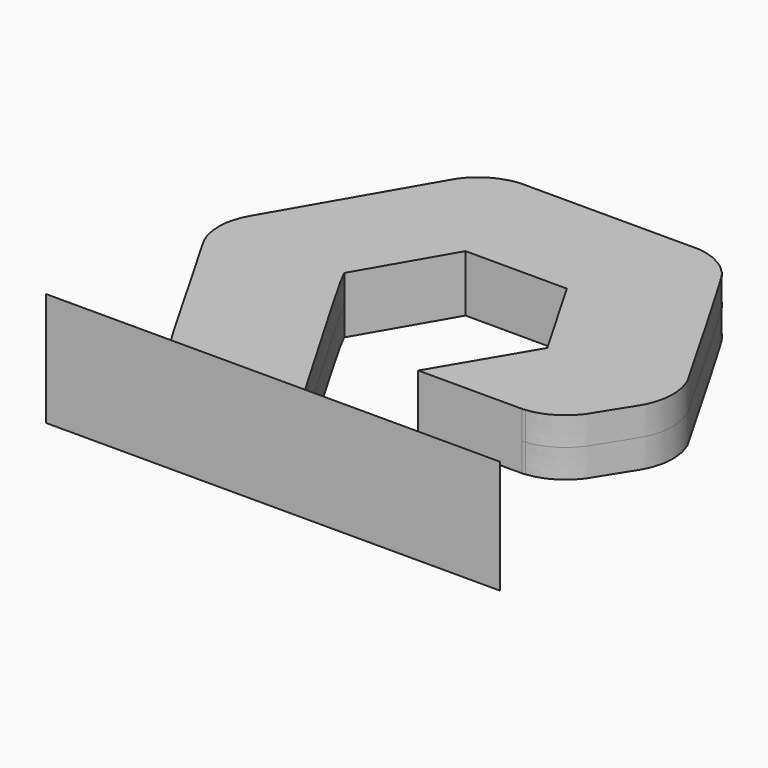
from build123d import *

# Parameters (mm, degrees)
F1_DEPTH    = 3.175
F2_DEPTH    = 1.5875
F3_DEPTH    = 1.5875
F4_T1_DEPTH = 22.6801869736
F4_T3_DEPTH = 41.7253830583


# Not quite as in the source:
# - a fillet or chamfer that OpenCascade refuses, or shapes differently, is made with other operations: its cross-section is extruded or revolved along the edge and cut away or added


with BuildPart() as f1:
    # F0 (on Top) → F1 (new body, symmetric)
    with BuildSketch(Plane.XY):
        with BuildLine():
            add(Edge.make_bspline(
                [(-8.0979492671, -8.4599665572), (-7.8144543772, -8.9512922446), (-7.4012331652, -9.6478596679), (-7.2094447017, -9.853233929), (-7.0198074368, -10.0624663427), (-6.8247908118, -10.2363901293), (-6.6355575508, -10.3900701529), (-6.4438841868, -10.5234739102), (-6.0350828964, -10.7264789939), (-5.8763022274, -10.78836422), (-5.4940772788, -10.9232334645), (-5.1611591338, -10.9716922009), (-4.9454318311, -10.9894729499), (-4.8368193396, -10.9980083466), (-1.8185705834, -10.9990381649), (0.9024133324, -10.9999665572)],
                knots=[0.5399683447, 0.5399683447, 0.5399683447, 0.5399683447, 0.583735527, 0.615598334, 0.6417416026, 0.6683965868, 0.6934366825, 0.7191935337, 0.7535274628, 0.7758085206, 0.8081226598, 0.8394404995, 0.861841058, 0.8754482187, 1, 1, 1, 1], degree=3))
            Line((-8.0979492671, -8.4599665572), (-12.7, -8.4599665572))
            Line((-12.7, -8.4599665572), (-12.7, -11.6349665572))
            Line((-12.7, -11.6349665572), (12.6951960847, -11.6349665572))
            Line((12.6951960847, -11.6349665572), (12.6951960847, -8.4599665572))
            Line((12.6951960847, -8.4599665572), (-0.5820742577, -8.4599665572))
            add(Edge.make_bspline(
                [(-0.5820742577, -8.4599665572), (-0.0948763272, -9.2939885426), (0.4037685026, -10.1469775499), (0.9024133324, -10.9999665572)],
                knots=[0.8523529488, 0.8523529488, 0.8523529488, 0.8523529488, 1, 1, 1, 1], degree=3))
        make_face()
        with BuildLine():
            Line((-0.5820742577, -8.4599665572), (-8.0979492671, -8.4599665572))
            add(Edge.make_bspline(
                [(-8.0979492671, -8.4599665572), (-7.8144543772, -8.9512922446), (-7.4012331652, -9.6478596679), (-7.2094447017, -9.853233929), (-7.0198074368, -10.0624663427), (-6.8247908118, -10.2363901293), (-6.6355575508, -10.3900701529), (-6.4438841868, -10.5234739102), (-6.0350828964, -10.7264789939), (-5.8763022274, -10.78836422), (-5.4940772788, -10.9232334645), (-5.1611591338, -10.9716922009), (-4.9454318311, -10.9894729499), (-4.8368193396, -10.9980083466), (-1.8185705834, -10.9990381649), (0.9024133324, -10.9999665572)],
                knots=[0.5399683447, 0.5399683447, 0.5399683447, 0.5399683447, 0.583735527, 0.615598334, 0.6417416026, 0.6683965868, 0.6934366825, 0.7191935337, 0.7535274628, 0.7758085206, 0.8081226598, 0.8394404995, 0.861841058, 0.8754482187, 1, 1, 1, 1], degree=3))
            add(Edge.make_bspline(
                [(-0.5820742577, -8.4599665572), (-0.0948763272, -9.2939885426), (0.4037685026, -10.1469775499), (0.9024133324, -10.9999665572)],
                knots=[0.8523529488, 0.8523529488, 0.8523529488, 0.8523529488, 1, 1, 1, 1], degree=3))
        make_face()
    extrude(amount=F1_DEPTH, both=True)

    # F0 (on Top) → F2 (cut, symmetric)
    with BuildSketch(Plane.XY):
        with BuildLine():
            add(Edge.make_bspline(
                [(-4.9467352219, 11.8727972619), (-2.6941970372, 11.8727972619), (-0.4416588525, 11.8727972619), (1.8108793323, 11.8727972619)],
                knots=[0.5524163134, 0.5524163134, 0.5524163134, 0.5524163134, 7.3100308676, 7.3100308676, 7.3100308676, 7.3100308676], degree=3))
            add(Edge.make_bspline(
                [(-12.1819954365, 2.2322773002), (-10.2153621206, 5.6292283823), (-7.918654142, 9.5963149713), (-7.7561059918, 9.8938723276), (-7.595936966, 10.1748103574), (-7.4488921306, 10.429639936), (-7.2380091716, 10.7143793357), (-7.0022497381, 10.9732635429), (-6.7468930063, 11.1814042046), (-6.6123462397, 11.2802086076), (-6.44534623, 11.390971666), (-6.3180815613, 11.463666659), (-6.1526142879, 11.5500745414), (-6.0434056072, 11.6051608595), (-5.8991320293, 11.660363592), (-5.6381957934, 11.7542790581), (-5.4211920209, 11.8110346891), (-5.1249038455, 11.8530818861), (-5.1009011539, 11.8676549492), (-4.9467352219, 11.8727972619)],
                knots=[0, 0, 0, 0, 0.1520022985, 0.1775139721, 0.2052814017, 0.2338919375, 0.2644870562, 0.2956347735, 0.3249719317, 0.3463123249, 0.3689682109, 0.3892301717, 0.411329997, 0.4293235674, 0.449497138, 0.4765503291, 0.5022012755, 0.5278147587, 0.5520405652, 0.5520405652, 0.5520405652, 0.5520405652], degree=3))
            add(Edge.make_bspline(
                [(-12.1819954365, 2.2322773002), (-12.2139037883, 2.1703194424), (-12.283482926, 2.0352145533), (-12.4406884255, 1.7801306072), (-12.6198918883, 1.2441500466), (-12.7164267868, 0.7551726738), (-12.7062312963, 0.3123164438), (-12.6510102494, -0.2863243011), (-12.5128439568, -0.6906531958), (-12.348735221, -1.0976190794), (-11.6470462247, -2.2552827891), (-11.0471565611, -3.3365181876), (-9.6670924889, -5.6885534643), (-8.4674528036, -7.819579074), (-8.0979492671, -8.4599665572)],
                knots=[0, 0, 0, 0, 0.0239021006, 0.0521207603, 0.0910959498, 0.1277402468, 0.1623042864, 0.2023672629, 0.23552051, 0.2695660314, 0.3281617082, 0.3861383143, 0.4829227709, 0.5399683447, 0.5399683447, 0.5399683447, 0.5399683447], degree=3))
            Line((-8.0979492671, -8.4599665572), (-0.5820742577, -8.4599665572))
            add(Edge.make_bspline(
                [(-5.6781647727, 0.4474149318), (-5.6798237666, 0.4432516249), (-5.716895521, 0.3502186819), (-3.2687593621, -3.8606973389), (-0.5820742577, -8.4599665572)],
                knots=[0, 0, 0, 0, 0.0381435521, 0.8523529488, 0.8523529488, 0.8523529488, 0.8523529488], degree=3))
            add(Edge.make_bspline(
                [(-2.836742904, 5.3628673777), (-3.7838835269, 3.7243832291), (-4.7310241498, 2.0858990805), (-5.6781647727, 0.4474149318)],
                knots=[0, 0, 0, 0, 5.6776184253, 5.6776184253, 5.6776184253, 5.6776184253], degree=3))
            add(Edge.make_bspline(
                [(2.8362337034, 5.3595150821), (0.9452415009, 5.360632514), (-0.9457507016, 5.3617499458), (-2.836742904, 5.3628673777)],
                knots=[0, 0, 0, 0, 5.6729775979, 5.6729775979, 5.6729775979, 5.6729775979], degree=3))
            add(Edge.make_bspline(
                [(5.6763379835, 0.4443899379), (4.7296365568, 2.082764986), (3.7829351301, 3.721140034), (2.8362337034, 5.3595150821)],
                knots=[0, 0, 0, 0, 5.6766757442, 5.6766757442, 5.6766757442, 5.6766757442], degree=3))
            add(Edge.make_bspline(
                [(2.6081528049, -4.7463672236), (3.6308811978, -3.0161148364), (4.6536095906, -1.2858624492), (5.6763379835, 0.4443899379)],
                knots=[0, 0, 0, 0, 6.0297363292, 6.0297363292, 6.0297363292, 6.0297363292], degree=3))
            Line((2.6081528049, -4.7463672236), (8.3983913064, -4.7463672236))
            add(Edge.make_bspline(
                [(8.3983913064, -4.7463672236), (8.4285802649, -4.7476342502), (8.4896773359, -4.7501984863), (8.5516653278, -4.7371940519), (8.5830241442, -4.7306152992)],
                knots=[0, 0, 0, 0, 0.4941146609, 1, 1, 1, 1], degree=3))
            add(Edge.make_bspline(
                [(7.394594606, 10.4755461216), (7.4049946498, 10.4644086633), (7.4978359113, 10.3649844979), (12.37583426, 1.9246802289), (12.3732313137, 1.8788009391), (12.4554314204, 1.7100351498), (12.5092309984, 1.5407375676), (12.579223391, 1.3481749221), (12.6327811924, 1.1548508933), (12.6617328431, 0.9474132467), (12.6887145756, 0.7331187902), (12.7057320419, 0.4773166934), (12.6885501549, 0.1892988959), (12.6579644324, -0.1503660031), (12.6047454763, -0.3551130001), (12.5476882015, -0.5689364186), (12.4644072913, -0.7996513773), (12.3592844301, -1.0395808564), (12.2025247276, -1.3122675142), (11.5798542764, -2.2842021351), (11.0022863487, -3.2119016224), (10.8931559285, -3.3988812592), (10.7117863794, -3.6224692911), (10.497630846, -3.8442513774), (10.2817003921, -4.0291717223), (10.0560553294, -4.2067210739), (9.8433649464, -4.3187164368), (9.7865197525, -4.3546553415), (9.5130416542, -4.505924573), (9.2077822138, -4.5905623978), (9.0144989656, -4.6706733119), (8.6495598585, -4.7218623963), (8.5981329416, -4.7286277074), (8.5830241442, -4.7306152992)],
                knots=[0, 0, 0, 0, 0.0211617068, 0.1889107002, 0.2086954298, 0.2296465529, 0.2530764843, 0.2773859957, 0.3015816681, 0.3261482383, 0.3512044462, 0.3783001026, 0.40768826, 0.4390979831, 0.4639315394, 0.4889953709, 0.5158573886, 0.5426802508, 0.5721507083, 0.6312181763, 0.6877344447, 0.7121562897, 0.7402266081, 0.7704940169, 0.7992541414, 0.828820597, 0.8543275782, 0.8684516809, 0.8979328023, 0.9286239977, 0.9544581079, 0.9866201736, 1, 1, 1, 1], degree=3))
            add(Edge.make_bspline(
                [(5.0841737539, 11.8727972619), (5.1354007842, 11.8660248609), (5.285102127, 11.8344246259), (5.511192311, 11.7972110307), (5.856974007, 11.6822825291), (6.0571511062, 11.6028524692), (6.5572225021, 11.3301125557), (6.8102335511, 11.1329565648), (7.0714115659, 10.8810767284), (7.2647332021, 10.6836819238), (7.3523685742, 10.5432240362), (7.394594606, 10.4755461216)],
                knots=[0.7441231562, 0.7441231562, 0.7441231562, 0.7441231562, 0.7668331465, 0.7924407066, 0.8229285687, 0.8479598314, 0.8863005426, 0.9166541286, 0.9473218688, 0.974617687, 1, 1, 1, 1], degree=3))
            add(Edge.make_bspline(
                [(4.7206622548, 11.8727972619), (4.8418327545, 11.8727972619), (4.9630032542, 11.8727972619), (5.0841737539, 11.8727972619)],
                knots=[10.2198137902, 10.2198137902, 10.2198137902, 10.2198137902, 10.5833252892, 10.5833252892, 10.5833252892, 10.5833252892], degree=3))
            add(Edge.make_bspline(
                [(1.8108793323, 11.8727972619), (3.1458171486, 11.8689304093), (4.2714307431, 11.8669693291), (4.7206622548, 11.8727972619)],
                knots=[0.6587883417, 0.6587883417, 0.6587883417, 0.6587883417, 0.7129256384, 0.7129256384, 0.7129256384, 0.7129256384], degree=3))
        make_face()
        with BuildLine():
            Line((-0.5820742577, -8.4599665572), (-8.0979492671, -8.4599665572))
            add(Edge.make_bspline(
                [(-8.0979492671, -8.4599665572), (-7.8144543772, -8.9512922446), (-7.4012331652, -9.6478596679), (-7.2094447017, -9.853233929), (-7.0198074368, -10.0624663427), (-6.8247908118, -10.2363901293), (-6.6355575508, -10.3900701529), (-6.4438841868, -10.5234739102), (-6.0350828964, -10.7264789939), (-5.8763022274, -10.78836422), (-5.4940772788, -10.9232334645), (-5.1611591338, -10.9716922009), (-4.9454318311, -10.9894729499), (-4.8368193396, -10.9980083466), (-1.8185705834, -10.9990381649), (0.9024133324, -10.9999665572)],
                knots=[0.5399683447, 0.5399683447, 0.5399683447, 0.5399683447, 0.583735527, 0.615598334, 0.6417416026, 0.6683965868, 0.6934366825, 0.7191935337, 0.7535274628, 0.7758085206, 0.8081226598, 0.8394404995, 0.861841058, 0.8754482187, 1, 1, 1, 1], degree=3))
            add(Edge.make_bspline(
                [(-0.5820742577, -8.4599665572), (-0.0948763272, -9.2939885426), (0.4037685026, -10.1469775499), (0.9024133324, -10.9999665572)],
                knots=[0.8523529488, 0.8523529488, 0.8523529488, 0.8523529488, 1, 1, 1, 1], degree=3))
        make_face()
    extrude(amount=F2_DEPTH, both=True, mode=Mode.SUBTRACT)

    # F4: chamfer of 3.175 on 4 edges, made by hand

    # F4_s2 → F4_t1 (cut)
    with BuildSketch(Plane.XY.offset(-11.3400934868)):
        Polygon((-9.525, -8.4599665572), (-12.7, -11.6349665572), (-12.7, -8.4599665572), align=None)
        Polygon((9.5201960847, -8.4599665572), (12.6951960847, -11.6349665572), (12.6951960847, -8.4599665572), align=None)
    extrude(amount=F4_T1_DEPTH, mode=Mode.SUBTRACT)

    # F4_s4 → F4_t3 (cut)
    with BuildSketch(Plane.YZ.offset(-20.8650934868)):
        Polygon((-8.4599665572, 0), (-11.6349665572, 3.175), (-8.4599665572, 3.175), align=None)
        Polygon((-8.4599665572, 0), (-11.6349665572, -3.175), (-8.4599665572, -3.175), align=None)
    extrude(amount=F4_T3_DEPTH, mode=Mode.SUBTRACT)


with BuildPart() as f3:
    # F0 (on Top) → F3 (new body, symmetric)
    with BuildSketch(Plane.XY):
        with BuildLine():
            add(Edge.make_bspline(
                [(-4.9467352219, 11.8727972619), (-2.6941970372, 11.8727972619), (-0.4416588525, 11.8727972619), (1.8108793323, 11.8727972619)],
                knots=[0.5524163134, 0.5524163134, 0.5524163134, 0.5524163134, 7.3100308676, 7.3100308676, 7.3100308676, 7.3100308676], degree=3))
            add(Edge.make_bspline(
                [(-12.1819954365, 2.2322773002), (-10.2153621206, 5.6292283823), (-7.918654142, 9.5963149713), (-7.7561059918, 9.8938723276), (-7.595936966, 10.1748103574), (-7.4488921306, 10.429639936), (-7.2380091716, 10.7143793357), (-7.0022497381, 10.9732635429), (-6.7468930063, 11.1814042046), (-6.6123462397, 11.2802086076), (-6.44534623, 11.390971666), (-6.3180815613, 11.463666659), (-6.1526142879, 11.5500745414), (-6.0434056072, 11.6051608595), (-5.8991320293, 11.660363592), (-5.6381957934, 11.7542790581), (-5.4211920209, 11.8110346891), (-5.1249038455, 11.8530818861), (-5.1009011539, 11.8676549492), (-4.9467352219, 11.8727972619)],
                knots=[0, 0, 0, 0, 0.1520022985, 0.1775139721, 0.2052814017, 0.2338919375, 0.2644870562, 0.2956347735, 0.3249719317, 0.3463123249, 0.3689682109, 0.3892301717, 0.411329997, 0.4293235674, 0.449497138, 0.4765503291, 0.5022012755, 0.5278147587, 0.5520405652, 0.5520405652, 0.5520405652, 0.5520405652], degree=3))
            add(Edge.make_bspline(
                [(-12.1819954365, 2.2322773002), (-12.2139037883, 2.1703194424), (-12.283482926, 2.0352145533), (-12.4406884255, 1.7801306072), (-12.6198918883, 1.2441500466), (-12.7164267868, 0.7551726738), (-12.7062312963, 0.3123164438), (-12.6510102494, -0.2863243011), (-12.5128439568, -0.6906531958), (-12.348735221, -1.0976190794), (-11.6470462247, -2.2552827891), (-11.0471565611, -3.3365181876), (-9.6670924889, -5.6885534643), (-8.4674528036, -7.819579074), (-8.0979492671, -8.4599665572)],
                knots=[0, 0, 0, 0, 0.0239021006, 0.0521207603, 0.0910959498, 0.1277402468, 0.1623042864, 0.2023672629, 0.23552051, 0.2695660314, 0.3281617082, 0.3861383143, 0.4829227709, 0.5399683447, 0.5399683447, 0.5399683447, 0.5399683447], degree=3))
            Line((-8.0979492671, -8.4599665572), (-0.5820742577, -8.4599665572))
            add(Edge.make_bspline(
                [(-5.6781647727, 0.4474149318), (-5.6798237666, 0.4432516249), (-5.716895521, 0.3502186819), (-3.2687593621, -3.8606973389), (-0.5820742577, -8.4599665572)],
                knots=[0, 0, 0, 0, 0.0381435521, 0.8523529488, 0.8523529488, 0.8523529488, 0.8523529488], degree=3))
            add(Edge.make_bspline(
                [(-2.836742904, 5.3628673777), (-3.7838835269, 3.7243832291), (-4.7310241498, 2.0858990805), (-5.6781647727, 0.4474149318)],
                knots=[0, 0, 0, 0, 5.6776184253, 5.6776184253, 5.6776184253, 5.6776184253], degree=3))
            add(Edge.make_bspline(
                [(2.8362337034, 5.3595150821), (0.9452415009, 5.360632514), (-0.9457507016, 5.3617499458), (-2.836742904, 5.3628673777)],
                knots=[0, 0, 0, 0, 5.6729775979, 5.6729775979, 5.6729775979, 5.6729775979], degree=3))
            add(Edge.make_bspline(
                [(5.6763379835, 0.4443899379), (4.7296365568, 2.082764986), (3.7829351301, 3.721140034), (2.8362337034, 5.3595150821)],
                knots=[0, 0, 0, 0, 5.6766757442, 5.6766757442, 5.6766757442, 5.6766757442], degree=3))
            add(Edge.make_bspline(
                [(2.6081528049, -4.7463672236), (3.6308811978, -3.0161148364), (4.6536095906, -1.2858624492), (5.6763379835, 0.4443899379)],
                knots=[0, 0, 0, 0, 6.0297363292, 6.0297363292, 6.0297363292, 6.0297363292], degree=3))
            Line((2.6081528049, -4.7463672236), (8.3983913064, -4.7463672236))
            add(Edge.make_bspline(
                [(8.3983913064, -4.7463672236), (8.4285802649, -4.7476342502), (8.4896773359, -4.7501984863), (8.5516653278, -4.7371940519), (8.5830241442, -4.7306152992)],
                knots=[0, 0, 0, 0, 0.4941146609, 1, 1, 1, 1], degree=3))
            add(Edge.make_bspline(
                [(7.394594606, 10.4755461216), (7.4049946498, 10.4644086633), (7.4978359113, 10.3649844979), (12.37583426, 1.9246802289), (12.3732313137, 1.8788009391), (12.4554314204, 1.7100351498), (12.5092309984, 1.5407375676), (12.579223391, 1.3481749221), (12.6327811924, 1.1548508933), (12.6617328431, 0.9474132467), (12.6887145756, 0.7331187902), (12.7057320419, 0.4773166934), (12.6885501549, 0.1892988959), (12.6579644324, -0.1503660031), (12.6047454763, -0.3551130001), (12.5476882015, -0.5689364186), (12.4644072913, -0.7996513773), (12.3592844301, -1.0395808564), (12.2025247276, -1.3122675142), (11.5798542764, -2.2842021351), (11.0022863487, -3.2119016224), (10.8931559285, -3.3988812592), (10.7117863794, -3.6224692911), (10.497630846, -3.8442513774), (10.2817003921, -4.0291717223), (10.0560553294, -4.2067210739), (9.8433649464, -4.3187164368), (9.7865197525, -4.3546553415), (9.5130416542, -4.505924573), (9.2077822138, -4.5905623978), (9.0144989656, -4.6706733119), (8.6495598585, -4.7218623963), (8.5981329416, -4.7286277074), (8.5830241442, -4.7306152992)],
                knots=[0, 0, 0, 0, 0.0211617068, 0.1889107002, 0.2086954298, 0.2296465529, 0.2530764843, 0.2773859957, 0.3015816681, 0.3261482383, 0.3512044462, 0.3783001026, 0.40768826, 0.4390979831, 0.4639315394, 0.4889953709, 0.5158573886, 0.5426802508, 0.5721507083, 0.6312181763, 0.6877344447, 0.7121562897, 0.7402266081, 0.7704940169, 0.7992541414, 0.828820597, 0.8543275782, 0.8684516809, 0.8979328023, 0.9286239977, 0.9544581079, 0.9866201736, 1, 1, 1, 1], degree=3))
            add(Edge.make_bspline(
                [(5.0841737539, 11.8727972619), (5.1354007842, 11.8660248609), (5.285102127, 11.8344246259), (5.511192311, 11.7972110307), (5.856974007, 11.6822825291), (6.0571511062, 11.6028524692), (6.5572225021, 11.3301125557), (6.8102335511, 11.1329565648), (7.0714115659, 10.8810767284), (7.2647332021, 10.6836819238), (7.3523685742, 10.5432240362), (7.394594606, 10.4755461216)],
                knots=[0.7441231562, 0.7441231562, 0.7441231562, 0.7441231562, 0.7668331465, 0.7924407066, 0.8229285687, 0.8479598314, 0.8863005426, 0.9166541286, 0.9473218688, 0.974617687, 1, 1, 1, 1], degree=3))
            add(Edge.make_bspline(
                [(4.7206622548, 11.8727972619), (4.8418327545, 11.8727972619), (4.9630032542, 11.8727972619), (5.0841737539, 11.8727972619)],
                knots=[10.2198137902, 10.2198137902, 10.2198137902, 10.2198137902, 10.5833252892, 10.5833252892, 10.5833252892, 10.5833252892], degree=3))
            add(Edge.make_bspline(
                [(1.8108793323, 11.8727972619), (3.1458171486, 11.8689304093), (4.2714307431, 11.8669693291), (4.7206622548, 11.8727972619)],
                knots=[0.6587883417, 0.6587883417, 0.6587883417, 0.6587883417, 0.7129256384, 0.7129256384, 0.7129256384, 0.7129256384], degree=3))
        make_face()
        with BuildLine():
            Line((-0.5820742577, -8.4599665572), (-8.0979492671, -8.4599665572))
            add(Edge.make_bspline(
                [(-8.0979492671, -8.4599665572), (-7.8144543772, -8.9512922446), (-7.4012331652, -9.6478596679), (-7.2094447017, -9.853233929), (-7.0198074368, -10.0624663427), (-6.8247908118, -10.2363901293), (-6.6355575508, -10.3900701529), (-6.4438841868, -10.5234739102), (-6.0350828964, -10.7264789939), (-5.8763022274, -10.78836422), (-5.4940772788, -10.9232334645), (-5.1611591338, -10.9716922009), (-4.9454318311, -10.9894729499), (-4.8368193396, -10.9980083466), (-1.8185705834, -10.9990381649), (0.9024133324, -10.9999665572)],
                knots=[0.5399683447, 0.5399683447, 0.5399683447, 0.5399683447, 0.583735527, 0.615598334, 0.6417416026, 0.6683965868, 0.6934366825, 0.7191935337, 0.7535274628, 0.7758085206, 0.8081226598, 0.8394404995, 0.861841058, 0.8754482187, 1, 1, 1, 1], degree=3))
            add(Edge.make_bspline(
                [(-0.5820742577, -8.4599665572), (-0.0948763272, -9.2939885426), (0.4037685026, -10.1469775499), (0.9024133324, -10.9999665572)],
                knots=[0.8523529488, 0.8523529488, 0.8523529488, 0.8523529488, 1, 1, 1, 1], degree=3))
        make_face()
    extrude(amount=F3_DEPTH, both=True)


solid = Compound([f1.part, f3.part])
